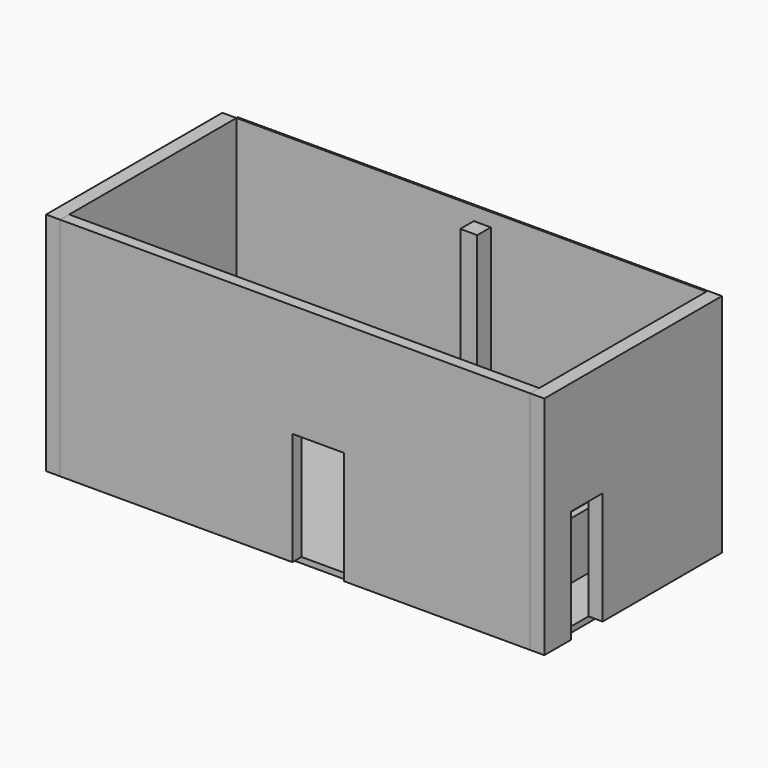
from build123d import *

# Parameters (mm, degrees)
F1_W      = 8320
F1_H      = 3700
F2_DEPTH  = 100
F3_W      = 300
F3_H      = 300
F4_DEPTH  = 4000
F3_W_2    = 280
F3_H_2    = 310
F3_W_3    = 310
F5_DEPTH  = 500
F3_W_4    = 120
F3_H_3    = 2400
F6_DEPTH  = 1010
F8_DEPTH  = 4000
F9_DEPTH  = 4000
F10_DEPTH = 4000
F7_W      = 8320
F7_H      = 200
F11_DEPTH = 4000
F12_W     = 700
F12_H     = 2000
F13_DEPTH = 8820.001
F14_W     = 900
F14_H     = 2000
F15_DEPTH = 8820.001
F16_W     = 910
F16_H     = 2000
F17_DEPTH = 3930.001


with BuildPart() as f2:
    # F1 (on Top) → F2 (new body)
    with BuildSketch(Plane.XY):
        Rectangle(F1_W, F1_H)
    extrude(amount=-F2_DEPTH)

    # F3 (on face) → F4 (join)
    with BuildSketch(Plane.XY):
        with Locations((480, 1340)):
            Rectangle(F3_W, F3_H)
    extrude(amount=F4_DEPTH)

    # F3 (on face) → F5 (join)
    with BuildSketch(Plane.XY):
        with Locations((-3100, 1695)):
            Rectangle(F3_W_2, F3_H_2)
        with Locations((-840, 1695)):
            Rectangle(F3_W_2, F3_H_2)
        with Locations((2285, 1695)):
            Rectangle(F3_W_3, F3_H_2)
        with Locations((485.2361369133, 1695)):
            Rectangle(F3_W_3, F3_H_2)
    extrude(amount=F5_DEPTH)

    # F3 (on face) → F6 (join)
    with BuildSketch(Plane.XY):
        with Locations((3290, 650)):
            Rectangle(F3_W_4, F3_H_3)
    extrude(amount=F6_DEPTH)


with BuildPart() as f8:
    # F7 (on face) → F8 (new body)
    with BuildSketch(Plane.XY):
        Polygon((-4160, 1880), (-4160, 1850), (-3240, 1850), (-2960, 1850), (-980, 1850), (-700, 1850), (330.2361369133, 1850), (640.2361369133, 1850), (2130, 1850), (2440, 1850), (3230, 1850), (3350, 1850), (4160, 1850), (4160, 1880), align=None)
    extrude(amount=F8_DEPTH)


with BuildPart() as f9:
    # F7 (on face) → F9 (new body)
    with BuildSketch(Plane.XY):
        Polygon((4410, 1880), (4160, 1880), (4160, 1850), (4160, -1850), (4160, -2050), (4410, -2050), align=None)
    extrude(amount=F9_DEPTH)

    # F12 (on face) → F13 (cut, through all)
    with BuildSketch(Plane.YZ.offset(4410)):
        with Locations((-1110, 1000)):
            Rectangle(F12_W, F12_H)
    extrude(amount=-F13_DEPTH, mode=Mode.SUBTRACT)


with BuildPart() as f10:
    # F7 (on face) → F10 (new body)
    with BuildSketch(Plane.XY):
        Polygon((-4160, -1850), (-4160, 1850), (-4410, 1850), (-4410, -2050), (-4160, -2050), align=None)
    extrude(amount=F10_DEPTH)

    # F14 (on face) → F15 (cut, through all)
    with BuildSketch(Plane(origin=(-4410, 0, 0), x_dir=(0, -1, 0), z_dir=(-1, 0, 0))):
        with Locations((560, 1000)):
            Rectangle(F14_W, F14_H)
    extrude(amount=-F15_DEPTH, mode=Mode.SUBTRACT)


with BuildPart() as f11:
    # F7 (on face) → F11 (new body)
    with BuildSketch(Plane.XY):
        with Locations((0, -1950)):
            Rectangle(F7_W, F7_H)
    extrude(amount=F11_DEPTH)

    # F16 (on face) → F17 (cut, through all)
    with BuildSketch(Plane.XZ.offset(2050)):
        with Locations((405, 1000)):
            Rectangle(F16_W, F16_H)
    extrude(amount=-F17_DEPTH, mode=Mode.SUBTRACT)


solid = Compound([f2.part, f8.part, f9.part, f10.part, f11.part])
